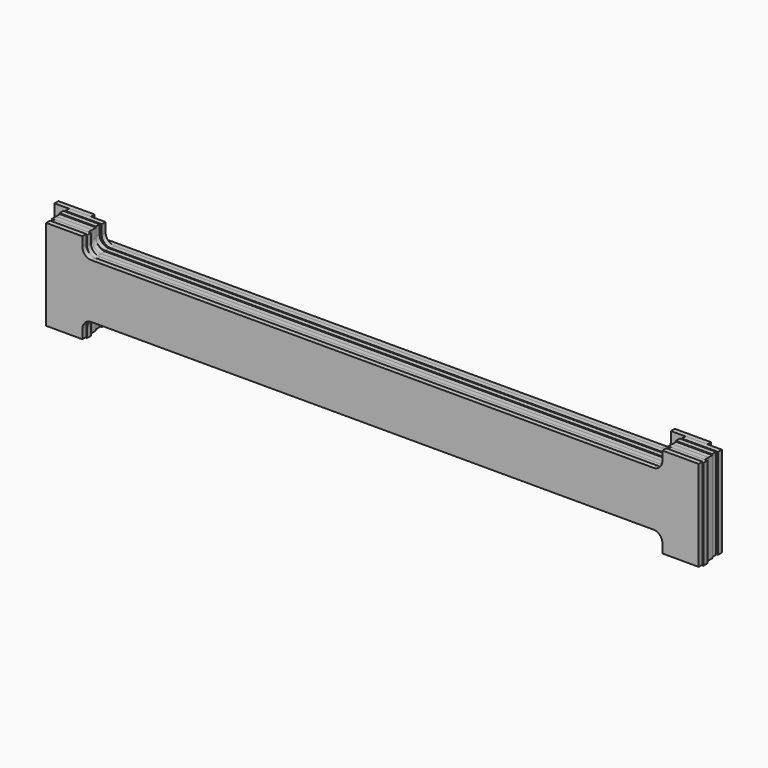
from build123d import *

# Parameters (mm, degrees)
F1_DEPTH  = 0.27
F4_DEPTH  = 0.27
F7_DEPTH  = 0.27
F10_DEPTH = 0.27
F13_DEPTH = 0.27
F14_DEPTH = 0.27
F15_DEPTH = 0.27
F18_DEPTH = 0.27
F21_DEPTH = 0.27


with BuildPart() as f1:
    # F0 (on Front) → F1 (new body)
    with BuildSketch(Plane.XZ):
        with BuildLine():
            Line((-16, 2.5), (-18, 2.5))
            Line((-18, 2.5), (-18, 0))
            Line((-18, 0), (18, 0))
            Line((18, 0), (18, 2.5))
            Line((18, 2.5), (16, 2.5))
            Line((16, 2.5), (16, 2))
            ThreePointArc((16, 2), (15.8535533906, 1.6464466094), (15.5, 1.5))
            Line((15.5, 1.5), (0, 1.5))
            Line((0, 1.5), (-15.5, 1.5))
            ThreePointArc((-15.5, 1.5), (-15.8535533906, 1.6464466094), (-16, 2))
            Line((-16, 2), (-16, 2.5))
        make_face()
        with BuildLine():
            Line((18, 0), (-18, 0))
            Line((-18, 0), (-18, -2.5))
            Line((-18, -2.5), (-16, -2.5))
            Line((-16, -2.5), (-16, -2))
            ThreePointArc((-16, -2), (-15.8535533906, -1.6464466094), (-15.5, -1.5))
            Line((-15.5, -1.5), (0, -1.5))
            Line((0, -1.5), (15.5, -1.5))
            ThreePointArc((15.5, -1.5), (15.8535533906, -1.6464466094), (16, -2))
            Line((16, -2), (16, -2.5))
            Line((16, -2.5), (18, -2.5))
            Line((18, -2.5), (18, 0))
        make_face()
    extrude(amount=F1_DEPTH)

    # F3 (on offset) → F4 (cut)
    with BuildSketch(Plane.XZ.offset(0.27)):
        with BuildLine():
            Line((-15.1841846166, 2.5122108632), (-17.1841846166, 2.5122108632))
            Line((-17.1841846166, 2.5122108632), (-17.1841846166, 0.0122108632))
            Line((-17.1841846166, 0.0122108632), (18.8158153834, 0.0122108632))
            Line((18.8158153834, 0.0122108632), (18.8158153834, 2.5122108632))
            Line((18.8158153834, 2.5122108632), (16.8158153834, 2.5122108632))
            Line((16.8158153834, 2.5122108632), (16.8158153834, 2.0122108632))
            ThreePointArc((16.8158153834, 2.0122108632), (16.669368774, 1.6586574726), (16.3158153834, 1.5122108632))
            Line((16.3158153834, 1.5122108632), (0.8158153834, 1.5122108632))
            Line((0.8158153834, 1.5122108632), (-14.6841846166, 1.5122108632))
            ThreePointArc((-14.6841846166, 1.5122108632), (-15.0377380072, 1.6586574726), (-15.1841846166, 2.0122108632))
            Line((-15.1841846166, 2.0122108632), (-15.1841846166, 2.5122108632))
        make_face()
        with BuildLine():
            Line((18.8158153834, 0.0122108632), (-17.1841846166, 0.0122108632))
            Line((-17.1841846166, 0.0122108632), (-17.1841846166, -2.4877891368))
            Line((-17.1841846166, -2.4877891368), (-15.1841846166, -2.4877891368))
            Line((-15.1841846166, -2.4877891368), (-15.1841846166, -1.9877891368))
            ThreePointArc((-15.1841846166, -1.9877891368), (-15.0377380072, -1.6342357462), (-14.6841846166, -1.4877891368))
            Line((-14.6841846166, -1.4877891368), (0.8158153834, -1.4877891368))
            Line((0.8158153834, -1.4877891368), (16.3158153834, -1.4877891368))
            ThreePointArc((16.3158153834, -1.4877891368), (16.669368774, -1.6342357462), (16.8158153834, -1.9877891368))
            Line((16.8158153834, -1.9877891368), (16.8158153834, -2.4877891368))
            Line((16.8158153834, -2.4877891368), (18.8158153834, -2.4877891368))
            Line((18.8158153834, -2.4877891368), (18.8158153834, 0.0122108632))
        make_face()
    extrude(amount=F4_DEPTH, mode=Mode.SUBTRACT)

    # F9 (on offset) → F10 (cut)
    with BuildSketch(Plane.XZ.offset(0.81)):
        with BuildLine():
            Line((-15.2458471914, 2.4499582283), (-17.2458471914, 2.4499582283))
            Line((-17.2458471914, 2.4499582283), (-17.2458471914, -0.0500417717))
            Line((-17.2458471914, -0.0500417717), (18.7541528086, -0.0500417717))
            Line((18.7541528086, -0.0500417717), (18.7541528086, 2.4499582283))
            Line((18.7541528086, 2.4499582283), (16.7541528086, 2.4499582283))
            Line((16.7541528086, 2.4499582283), (16.7541528086, 1.9499582283))
            ThreePointArc((16.7541528086, 1.9499582283), (16.6077061992, 1.5964048377), (16.2541528086, 1.4499582283))
            Line((16.2541528086, 1.4499582283), (0.7541528086, 1.4499582283))
            Line((0.7541528086, 1.4499582283), (-14.7458471914, 1.4499582283))
            ThreePointArc((-14.7458471914, 1.4499582283), (-15.099400582, 1.5964048377), (-15.2458471914, 1.9499582283))
            Line((-15.2458471914, 1.9499582283), (-15.2458471914, 2.4499582283))
        make_face()
        with BuildLine():
            Line((18.7541528086, -0.0500417717), (-17.2458471914, -0.0500417717))
            Line((-17.2458471914, -0.0500417717), (-17.2458471914, -2.5500417717))
            Line((-17.2458471914, -2.5500417717), (-15.2458471914, -2.5500417717))
            Line((-15.2458471914, -2.5500417717), (-15.2458471914, -2.0500417717))
            ThreePointArc((-15.2458471914, -2.0500417717), (-15.099400582, -1.6964883811), (-14.7458471914, -1.5500417717))
            Line((-14.7458471914, -1.5500417717), (0.7541528086, -1.5500417717))
            Line((0.7541528086, -1.5500417717), (16.2541528086, -1.5500417717))
            ThreePointArc((16.2541528086, -1.5500417717), (16.6077061992, -1.6964883811), (16.7541528086, -2.0500417717))
            Line((16.7541528086, -2.0500417717), (16.7541528086, -2.5500417717))
            Line((16.7541528086, -2.5500417717), (18.7541528086, -2.5500417717))
            Line((18.7541528086, -2.5500417717), (18.7541528086, -0.0500417717))
        make_face()
    extrude(amount=F10_DEPTH, mode=Mode.SUBTRACT)


with BuildPart() as f7:
    # F6 (on offset) → F7 (new body)
    with BuildSketch(Plane.XZ.offset(0.54)):
        with BuildLine():
            Line((-15.2949587338, 2.4747978128), (-17.2949587338, 2.4747978128))
            Line((-17.2949587338, 2.4747978128), (-17.2949587338, -0.0252021872))
            Line((-17.2949587338, -0.0252021872), (18.7050412662, -0.0252021872))
            Line((18.7050412662, -0.0252021872), (18.7050412662, 2.4747978128))
            Line((18.7050412662, 2.4747978128), (16.7050412662, 2.4747978128))
            Line((16.7050412662, 2.4747978128), (16.7050412662, 1.9747978128))
            ThreePointArc((16.7050412662, 1.9747978128), (16.5585946567, 1.6212444222), (16.2050412662, 1.4747978128))
            Line((16.2050412662, 1.4747978128), (0.7050412662, 1.4747978128))
            Line((0.7050412662, 1.4747978128), (-14.7949587338, 1.4747978128))
            ThreePointArc((-14.7949587338, 1.4747978128), (-15.1485121244, 1.6212444222), (-15.2949587338, 1.9747978128))
            Line((-15.2949587338, 1.9747978128), (-15.2949587338, 2.4747978128))
        make_face()
        with BuildLine():
            Line((18.7050412662, -0.0252021872), (-17.2949587338, -0.0252021872))
            Line((-17.2949587338, -0.0252021872), (-17.2949587338, -2.5252021872))
            Line((-17.2949587338, -2.5252021872), (-15.2949587338, -2.5252021872))
            Line((-15.2949587338, -2.5252021872), (-15.2949587338, -2.0252021872))
            ThreePointArc((-15.2949587338, -2.0252021872), (-15.1485121244, -1.6716487966), (-14.7949587338, -1.5252021872))
            Line((-14.7949587338, -1.5252021872), (0.7050412662, -1.5252021872))
            Line((0.7050412662, -1.5252021872), (16.2050412662, -1.5252021872))
            ThreePointArc((16.2050412662, -1.5252021872), (16.5585946567, -1.6716487966), (16.7050412662, -2.0252021872))
            Line((16.7050412662, -2.0252021872), (16.7050412662, -2.5252021872))
            Line((16.7050412662, -2.5252021872), (18.7050412662, -2.5252021872))
            Line((18.7050412662, -2.5252021872), (18.7050412662, -0.0252021872))
        make_face()
    extrude(amount=F7_DEPTH)


with BuildPart() as f13:
    # F12 (on offset) → F13 (new body)
    with BuildSketch(Plane.XZ.offset(1.08)):
        with BuildLine():
            Line((-15.2727272727, 2.4318181818), (-17.2727272727, 2.4318181818))
            Line((-17.2727272727, 2.4318181818), (-17.2727272727, -0.0681818182))
            Line((-17.2727272727, -0.0681818182), (18.7272727273, -0.0681818182))
            Line((18.7272727273, -0.0681818182), (18.7272727273, 2.4318181818))
            Line((18.7272727273, 2.4318181818), (16.7272727273, 2.4318181818))
            Line((16.7272727273, 2.4318181818), (16.7272727273, 1.9318181818))
            ThreePointArc((16.7272727273, 1.9318181818), (16.5808261179, 1.5782647912), (16.2272727273, 1.4318181818))
            Line((16.2272727273, 1.4318181818), (0.7272727273, 1.4318181818))
            Line((0.7272727273, 1.4318181818), (-14.7727272727, 1.4318181818))
            ThreePointArc((-14.7727272727, 1.4318181818), (-15.1262806633, 1.5782647912), (-15.2727272727, 1.9318181818))
            Line((-15.2727272727, 1.9318181818), (-15.2727272727, 2.4318181818))
        make_face()
        with BuildLine():
            Line((18.7272727273, -0.0681818182), (-17.2727272727, -0.0681818182))
            Line((-17.2727272727, -0.0681818182), (-17.2727272727, -2.5681818182))
            Line((-17.2727272727, -2.5681818182), (-15.2727272727, -2.5681818182))
            Line((-15.2727272727, -2.5681818182), (-15.2727272727, -2.0681818182))
            ThreePointArc((-15.2727272727, -2.0681818182), (-15.1262806633, -1.7146284276), (-14.7727272727, -1.5681818182))
            Line((-14.7727272727, -1.5681818182), (0.7272727273, -1.5681818182))
            Line((0.7272727273, -1.5681818182), (16.2272727273, -1.5681818182))
            ThreePointArc((16.2272727273, -1.5681818182), (16.5808261179, -1.7146284276), (16.7272727273, -2.0681818182))
            Line((16.7272727273, -2.0681818182), (16.7272727273, -2.5681818182))
            Line((16.7272727273, -2.5681818182), (18.7272727273, -2.5681818182))
            Line((18.7272727273, -2.5681818182), (18.7272727273, -0.0681818182))
        make_face()
    extrude(amount=F13_DEPTH)


with BuildPart() as f14:
    # F3 (on offset) → F14 (new body)
    with BuildSketch(Plane.XZ.offset(0.27)):
        with BuildLine():
            Line((-15.1841846166, 2.5122108632), (-17.1841846166, 2.5122108632))
            Line((-17.1841846166, 2.5122108632), (-17.1841846166, 0.0122108632))
            Line((-17.1841846166, 0.0122108632), (18.8158153834, 0.0122108632))
            Line((18.8158153834, 0.0122108632), (18.8158153834, 2.5122108632))
            Line((18.8158153834, 2.5122108632), (16.8158153834, 2.5122108632))
            Line((16.8158153834, 2.5122108632), (16.8158153834, 2.0122108632))
            ThreePointArc((16.8158153834, 2.0122108632), (16.669368774, 1.6586574726), (16.3158153834, 1.5122108632))
            Line((16.3158153834, 1.5122108632), (0.8158153834, 1.5122108632))
            Line((0.8158153834, 1.5122108632), (-14.6841846166, 1.5122108632))
            ThreePointArc((-14.6841846166, 1.5122108632), (-15.0377380072, 1.6586574726), (-15.1841846166, 2.0122108632))
            Line((-15.1841846166, 2.0122108632), (-15.1841846166, 2.5122108632))
        make_face()
        with BuildLine():
            Line((18.8158153834, 0.0122108632), (-17.1841846166, 0.0122108632))
            Line((-17.1841846166, 0.0122108632), (-17.1841846166, -2.4877891368))
            Line((-17.1841846166, -2.4877891368), (-15.1841846166, -2.4877891368))
            Line((-15.1841846166, -2.4877891368), (-15.1841846166, -1.9877891368))
            ThreePointArc((-15.1841846166, -1.9877891368), (-15.0377380072, -1.6342357462), (-14.6841846166, -1.4877891368))
            Line((-14.6841846166, -1.4877891368), (0.8158153834, -1.4877891368))
            Line((0.8158153834, -1.4877891368), (16.3158153834, -1.4877891368))
            ThreePointArc((16.3158153834, -1.4877891368), (16.669368774, -1.6342357462), (16.8158153834, -1.9877891368))
            Line((16.8158153834, -1.9877891368), (16.8158153834, -2.4877891368))
            Line((16.8158153834, -2.4877891368), (18.8158153834, -2.4877891368))
            Line((18.8158153834, -2.4877891368), (18.8158153834, 0.0122108632))
        make_face()
    extrude(amount=F14_DEPTH)


with BuildPart() as f15:
    # F12 (on offset) → F15 (new body)
    with BuildSketch(Plane.XZ.offset(1.08)):
        with BuildLine():
            Line((-15.2727272727, 2.4318181818), (-17.2727272727, 2.4318181818))
            Line((-17.2727272727, 2.4318181818), (-17.2727272727, -0.0681818182))
            Line((-17.2727272727, -0.0681818182), (18.7272727273, -0.0681818182))
            Line((18.7272727273, -0.0681818182), (18.7272727273, 2.4318181818))
            Line((18.7272727273, 2.4318181818), (16.7272727273, 2.4318181818))
            Line((16.7272727273, 2.4318181818), (16.7272727273, 1.9318181818))
            ThreePointArc((16.7272727273, 1.9318181818), (16.5808261179, 1.5782647912), (16.2272727273, 1.4318181818))
            Line((16.2272727273, 1.4318181818), (0.7272727273, 1.4318181818))
            Line((0.7272727273, 1.4318181818), (-14.7727272727, 1.4318181818))
            ThreePointArc((-14.7727272727, 1.4318181818), (-15.1262806633, 1.5782647912), (-15.2727272727, 1.9318181818))
            Line((-15.2727272727, 1.9318181818), (-15.2727272727, 2.4318181818))
        make_face()
        with BuildLine():
            Line((18.7272727273, -0.0681818182), (-17.2727272727, -0.0681818182))
            Line((-17.2727272727, -0.0681818182), (-17.2727272727, -2.5681818182))
            Line((-17.2727272727, -2.5681818182), (-15.2727272727, -2.5681818182))
            Line((-15.2727272727, -2.5681818182), (-15.2727272727, -2.0681818182))
            ThreePointArc((-15.2727272727, -2.0681818182), (-15.1262806633, -1.7146284276), (-14.7727272727, -1.5681818182))
            Line((-14.7727272727, -1.5681818182), (0.7272727273, -1.5681818182))
            Line((0.7272727273, -1.5681818182), (16.2272727273, -1.5681818182))
            ThreePointArc((16.2272727273, -1.5681818182), (16.5808261179, -1.7146284276), (16.7272727273, -2.0681818182))
            Line((16.7272727273, -2.0681818182), (16.7272727273, -2.5681818182))
            Line((16.7272727273, -2.5681818182), (18.7272727273, -2.5681818182))
            Line((18.7272727273, -2.5681818182), (18.7272727273, -0.0681818182))
        make_face()
    extrude(amount=-F15_DEPTH)


with BuildPart() as f18:
    # F17 (on offset) → F18 (new body)
    with BuildSketch(Plane.XZ.offset(1.35)):
        with BuildLine():
            Line((-15.1280487846, 2.4376975121), (-17.1280487846, 2.4376975121))
            Line((-17.1280487846, 2.4376975121), (-17.1280487846, -0.0623024879))
            Line((-17.1280487846, -0.0623024879), (18.8719512154, -0.0623024879))
            Line((18.8719512154, -0.0623024879), (18.8719512154, 2.4376975121))
            Line((18.8719512154, 2.4376975121), (16.8719512154, 2.4376975121))
            Line((16.8719512154, 2.4376975121), (16.8719512154, 1.9376975121))
            ThreePointArc((16.8719512154, 1.9376975121), (16.725504606, 1.5841441215), (16.3719512154, 1.4376975121))
            Line((16.3719512154, 1.4376975121), (0.8719512154, 1.4376975121))
            Line((0.8719512154, 1.4376975121), (-14.6280487846, 1.4376975121))
            ThreePointArc((-14.6280487846, 1.4376975121), (-14.9816021752, 1.5841441215), (-15.1280487846, 1.9376975121))
            Line((-15.1280487846, 1.9376975121), (-15.1280487846, 2.4376975121))
        make_face()
        with BuildLine():
            Line((18.8719512154, -0.0623024879), (-17.1280487846, -0.0623024879))
            Line((-17.1280487846, -0.0623024879), (-17.1280487846, -2.5623024879))
            Line((-17.1280487846, -2.5623024879), (-15.1280487846, -2.5623024879))
            Line((-15.1280487846, -2.5623024879), (-15.1280487846, -2.0623024879))
            ThreePointArc((-15.1280487846, -2.0623024879), (-14.9816021752, -1.7087490973), (-14.6280487846, -1.5623024879))
            Line((-14.6280487846, -1.5623024879), (0.8719512154, -1.5623024879))
            Line((0.8719512154, -1.5623024879), (16.3719512154, -1.5623024879))
            ThreePointArc((16.3719512154, -1.5623024879), (16.725504606, -1.7087490973), (16.8719512154, -2.0623024879))
            Line((16.8719512154, -2.0623024879), (16.8719512154, -2.5623024879))
            Line((16.8719512154, -2.5623024879), (18.8719512154, -2.5623024879))
            Line((18.8719512154, -2.5623024879), (18.8719512154, -0.0623024879))
        make_face()
    extrude(amount=F18_DEPTH)


with BuildPart() as f21:
    # F20 (on offset) → F21 (new body)
    with BuildSketch(Plane.XZ.offset(1.62)):
        with BuildLine():
            Line((-15.1708155028, 2.4804651617), (-17.1708155028, 2.4804651617))
            Line((-17.1708155028, 2.4804651617), (-17.1708155028, -0.0195348383))
            Line((-17.1708155028, -0.0195348383), (18.8291844972, -0.0195348383))
            Line((18.8291844972, -0.0195348383), (18.8291844972, 2.4804651617))
            Line((18.8291844972, 2.4804651617), (16.8291844972, 2.4804651617))
            Line((16.8291844972, 2.4804651617), (16.8291844972, 1.9804651617))
            ThreePointArc((16.8291844972, 1.9804651617), (16.6827378878, 1.6269117711), (16.3291844972, 1.4804651617))
            Line((16.3291844972, 1.4804651617), (0.8291844972, 1.4804651617))
            Line((0.8291844972, 1.4804651617), (-14.6708155028, 1.4804651617))
            ThreePointArc((-14.6708155028, 1.4804651617), (-15.0243688934, 1.6269117711), (-15.1708155028, 1.9804651617))
            Line((-15.1708155028, 1.9804651617), (-15.1708155028, 2.4804651617))
        make_face()
        with BuildLine():
            Line((18.8291844972, -0.0195348383), (-17.1708155028, -0.0195348383))
            Line((-17.1708155028, -0.0195348383), (-17.1708155028, -2.5195348383))
            Line((-17.1708155028, -2.5195348383), (-15.1708155028, -2.5195348383))
            Line((-15.1708155028, -2.5195348383), (-15.1708155028, -2.0195348383))
            ThreePointArc((-15.1708155028, -2.0195348383), (-15.0243688934, -1.6659814477), (-14.6708155028, -1.5195348383))
            Line((-14.6708155028, -1.5195348383), (0.8291844972, -1.5195348383))
            Line((0.8291844972, -1.5195348383), (16.3291844972, -1.5195348383))
            ThreePointArc((16.3291844972, -1.5195348383), (16.6827378878, -1.6659814477), (16.8291844972, -2.0195348383))
            Line((16.8291844972, -2.0195348383), (16.8291844972, -2.5195348383))
            Line((16.8291844972, -2.5195348383), (18.8291844972, -2.5195348383))
            Line((18.8291844972, -2.5195348383), (18.8291844972, -0.0195348383))
        make_face()
    extrude(amount=F21_DEPTH)


solid = Compound([f1.part, f7.part, f13.part, f14.part, f15.part, f18.part, f21.part])
